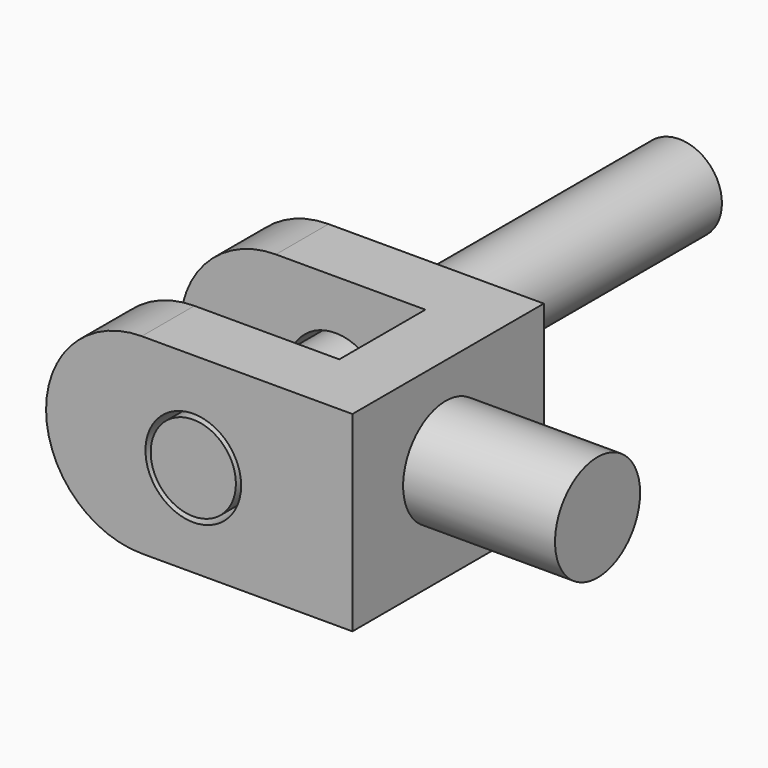
from build123d import *

# Parameters (mm, degrees)
F1_DEPTH  = 32
F2_R      = 8
F3_DEPTH  = 25.4
F4_R      = 8
F5_DEPTH  = 25.4
F6_R      = 16
F7_R      = 15.99999
F8_R      = 16
F9_R      = 15.99999
F10_R     = 8.8894259747
F11_DEPTH = 25.4
F12_R     = 7.125734637
F13_DEPTH = 101.6


# Not quite as in the source:
# - a fillet or chamfer is up to 0.001 mm smaller than in the source, because OpenCascade refuses the exact size


with BuildPart() as f1:
    # F0 (on Top) → F1 (new body)
    with BuildSketch(Plane.XY):
        Polygon((15.5333588993, 29), (-36.4666411007, 29), (-36.4666411007, 18), (4.5333588993, 18), (4.5333588993, 0), (-35.6989217131, 0), (-35.6989217131, -11), (15.5333588993, -11), align=None)
    extrude(amount=F1_DEPTH)

    # F2 (on face) → F3 (cut)
    with BuildSketch(Plane.XZ.offset(11)):
        with Locations((-11.0805211589, 15.3976073489)):
            Circle(F2_R)
    extrude(amount=-F3_DEPTH, mode=Mode.SUBTRACT)

    # F4 (on face) → F5 (cut)
    with BuildSketch(Plane(origin=(0, 29, 0), x_dir=(-1, 0, 0), z_dir=(0, 1, 0))):
        with Locations((10.5049097911, 15.6854130328)):
            Circle(F4_R)
    extrude(amount=-F5_DEPTH, mode=Mode.SUBTRACT)

    # F6
    f6_edges = [f1.edges().sort_by_distance(p)[0] for p in [
        (-35.698922, -5.5, 32),
    ]]
    fillet(f6_edges, radius=F6_R)

    # F7 (radius 16 in the source; OpenCascade refuses exactly that, so slightly less here)
    f7_edges = [f1.edges().sort_by_distance(p)[0] for p in [
        (-35.698922, -5.5, 0),
    ]]
    fillet(f7_edges, radius=F7_R)

    # F8
    f8_edges = [f1.edges().sort_by_distance(p)[0] for p in [
        (-36.466641, 23.5, 32),
    ]]
    fillet(f8_edges, radius=F8_R)

    # F9 (radius 16 in the source; OpenCascade refuses exactly that, so slightly less here)
    f9_edges = [f1.edges().sort_by_distance(p)[0] for p in [
        (-36.466641, 23.5, 0),
    ]]
    fillet(f9_edges, radius=F9_R)

    # F10 (on face) → F11 (join)
    with BuildSketch(Plane.YZ.offset(15.5333588993)):
        with Locations((8.4902700037, 17.1244423836)):
            Circle(F10_R)
    extrude(amount=F11_DEPTH)


with BuildPart() as f13:
    # F12 (on face) → F13 (new body)
    with BuildSketch(Plane.XZ.offset(11)):
        with Locations((-11.0805211589, 15.3976073489)):
            Circle(F12_R)
    extrude(amount=-F13_DEPTH)


solid = Compound([f1.part, f13.part])
